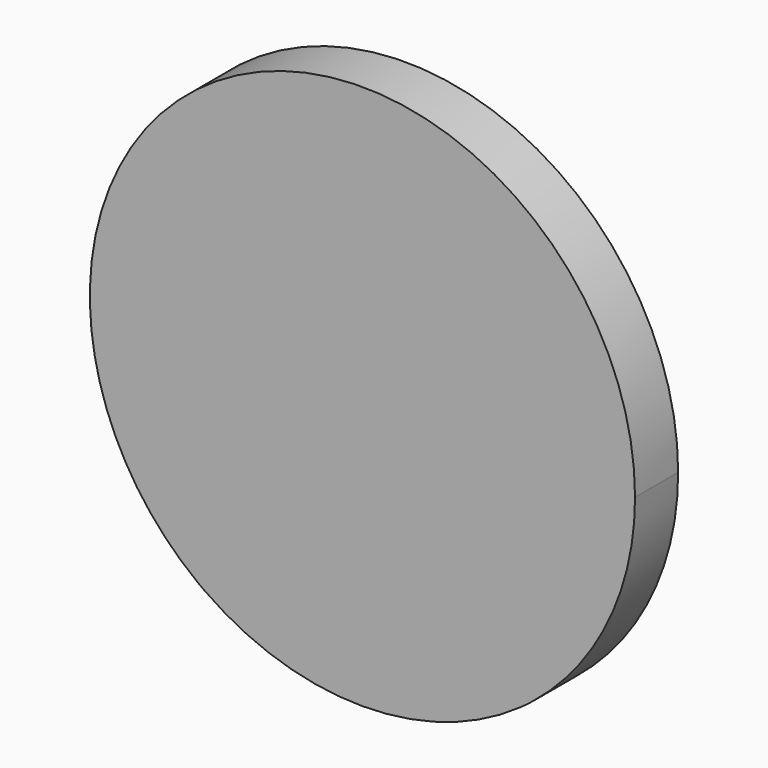
from build123d import *

# Parameters (mm, degrees)
F1_DEPTH = 10


# Not quite as in the source:
# - a feature names something its author has since deleted; it is built from what else it names


with BuildPart() as f1:
    # F0 (on Front) → F1 (new body)
    with BuildSketch(Plane.XZ):
        with BuildLine():
            ThreePointArc((0, 12.4140736889), (4.3797238065, 11.6158187371), (8.1961939537, 9.3237133283))
            Line((8.1961939537, 9.3237133283), (21.0697077151, 23.9681876437))
            ThreePointArc((21.0697077151, 23.9681876437), (18.4530079812, 27.8283575749), (18.0439527664, 32.4738611241))
            Line((18.0439527664, 32.4738611241), (12.5602155062, 33.3932852461))
            Line((12.5602155062, 33.3932852461), (7.5710593451, 36.5340338213))
            ThreePointArc((7.5710593451, 36.5340338213), (4.3242109258, 33.4682836339), (0, 32.3538112298))
            Line((0, 32.3538112298), (0, 12.4140736889))
        make_face()
        with BuildLine():
            ThreePointArc((-7.9262057201, 9.554291624), (-4.2131665816, 11.6772622181), (0, 12.4140736889))
            Line((0, 12.4140736889), (0, 32.3538112298))
            ThreePointArc((0, 32.3538112298), (-4.3563302657, 33.4861038791), (-7.6099407791, 36.5963641019))
            Line((-7.6099407791, 36.5963641019), (-12.278520326, 33.7106778775))
            Line((-12.278520326, 33.7106778775), (-17.78879081, 33.0882026957))
            ThreePointArc((-17.78879081, 33.0882026957), (-17.7466642393, 32.5900633313), (-17.73260723, 32.0903435349))
            ThreePointArc((-17.73260723, 32.0903435349), (-18.5760333574, 28.310954716), (-20.9462636845, 25.2487405378))
            Line((-20.9462636845, 25.2487405378), (-7.9262057201, 9.554291624))
        make_face()
        with BuildLine():
            Line((-12.278520326, 33.7106778775), (-7.6099407791, 36.5963641019))
            ThreePointArc((-7.6099407791, 36.5963641019), (-8.921680068, 41.9636267042), (-6.8304445709, 47.0778130421))
            ThreePointArc((-6.8304445709, 47.0778130421), (-17.0260006599, 47.3423785206), (-24.8514976267, 40.8016632631))
            ThreePointArc((-24.8514976267, 40.8016632631), (-20.0657845476, 38.0934673525), (-17.78879081, 33.0882026957))
            Line((-17.78879081, 33.0882026957), (-12.278520326, 33.7106778775))
        make_face()
        with BuildLine():
            ThreePointArc((-6.8304445709, 47.0778130421), (-8.921680068, 41.9636267042), (-7.6099407791, 36.5963641019))
            Line((-7.6099407791, 36.5963641019), (0, 41.3001291454))
            ThreePointArc((0, 41.3001291454), (-2.9563177988, 44.7314932731), (-6.8304445709, 47.0778130421))
        make_face()
        with BuildLine():
            ThreePointArc((-6.8304445709, 47.0778130421), (-2.9563177988, 44.7314932731), (0, 41.3001291454))
            ThreePointArc((0, 41.3001291454), (2.9670877078, 44.7179968563), (6.8263210631, 47.0826843755))
            ThreePointArc((6.8263210631, 47.0826843755), (-0.0031911285, 50.2464464918), (-6.8304445709, 47.0778130421))
        make_face()
        with BuildLine():
            Line((0, 41.3001291454), (7.5710593451, 36.5340338213))
            ThreePointArc((7.5710593451, 36.5340338213), (8.5956299393, 38.8198569439), (8.9463179156, 41.3001291454))
            ThreePointArc((8.9463179156, 41.3001291454), (8.3996143563, 44.3795906098), (6.8263210631, 47.0826843755))
            ThreePointArc((6.8263210631, 47.0826843755), (2.9670877078, 44.7179968563), (0, 41.3001291454))
        make_face()
        with BuildLine():
            Line((0, 41.3001291454), (0, 32.3538112298))
            ThreePointArc((0, 32.3538112298), (4.3242109258, 33.4682836339), (7.5710593451, 36.5340338213))
            Line((7.5710593451, 36.5340338213), (0, 41.3001291454))
        make_face()
        with BuildLine():
            ThreePointArc((-7.6099407791, 36.5963641019), (-4.3563302657, 33.4861038791), (0, 32.3538112298))
            Line((0, 32.3538112298), (0, 41.3001291454))
            Line((0, 41.3001291454), (-7.6099407791, 36.5963641019))
        make_face()
        with BuildLine():
            ThreePointArc((36.4223056753, 29.9139118839), (45.9083800473, 20.8806963335), (46.4937895072, 7.7947540314))
            ThreePointArc((46.4937895072, 7.7947540314), (49.4692239822, 4.3915233547), (50.5414702125, 0))
            ThreePointArc((50.5414702125, 0), (49.3916524089, -4.5377847699), (46.2196804198, -7.9804821571))
            ThreePointArc((46.2196804198, -7.9804821571), (45.2541028323, -22.5688235592), (34.2624022156, -32.2090809466))
            ThreePointArc((34.2624022156, -32.2090809466), (34.2845647661, -32.5811281227), (34.291956159, -32.953761518))
            ThreePointArc((34.291956159, -32.953761518), (33.6295574849, -36.4193105223), (31.7357494034, -39.3962708606))
            ThreePointArc((31.7357494034, -39.3962708606), (45.6327545118, -21.8374829955), (50.5887729434, 0))
            ThreePointArc((50.5887729434, 0), (0.6523386875, 50.5845668377), (-50.5719492199, 1.3045689002))
            ThreePointArc((-50.5719492199, 1.3045689002), (-49.1901644057, 5.1967911583), (-46.3448391854, 8.1905927165))
            ThreePointArc((-46.3448391854, 8.1905927165), (-45.5368746407, 21.848912941), (-35.4561087337, 31.0998954179))
            ThreePointArc((-35.4561087337, 31.0998954179), (-32.6224058372, 38.6491093328), (-24.8514976267, 40.8016632631))
            ThreePointArc((-24.8514976267, 40.8016632631), (-17.0260006599, 47.3423785206), (-6.8304445709, 47.0778130421))
            ThreePointArc((-6.8304445709, 47.0778130421), (-0.0031911285, 50.2464464918), (6.8263210631, 47.0826843755))
            ThreePointArc((6.8263210631, 47.0826843755), (17.6788975714, 47.324411831), (25.7932452382, 40.1137106881))
            ThreePointArc((25.7932452382, 40.1137106881), (33.2437406928, 37.9811469414), (36.4791003688, 30.9391189367))
            ThreePointArc((36.4791003688, 30.9391189367), (36.4648908183, 30.425729431), (36.4223056753, 29.9139118839))
        make_face()
        with BuildLine():
            ThreePointArc((-46.3448391854, 8.1905927165), (-40.2671562667, 9.9229363025), (-34.3745943291, 7.6388702415))
            Line((-34.3745943291, 7.6388702415), (-29.0687931112, 14.021677727))
            Line((-29.0687931112, 14.021677727), (-27.8149031494, 23.2813171291))
            ThreePointArc((-27.8149031494, 23.2813171291), (-32.9795051289, 25.8770971269), (-35.4561087337, 31.0998954179))
            ThreePointArc((-35.4561087337, 31.0998954179), (-45.5368746407, 21.848912941), (-46.3448391854, 8.1905927165))
        make_face()
        with BuildLine():
            ThreePointArc((-35.4561087337, 31.0998954179), (-32.9795051289, 25.8770971269), (-27.8149031494, 23.2813171291))
            Line((-27.8149031494, 23.2813171291), (-26.6220327467, 32.0903435349))
            ThreePointArc((-26.6220327467, 32.0903435349), (-31.1003542851, 32.1417240723), (-35.4561087337, 31.0998954179))
        make_face()
        with BuildLine():
            ThreePointArc((-35.4561087337, 31.0998954179), (-31.1003542851, 32.1417240723), (-26.6220327467, 32.0903435349))
            ThreePointArc((-26.6220327467, 32.0903435349), (-26.4240541647, 36.5856916795), (-24.8514976267, 40.8016632631))
            ThreePointArc((-24.8514976267, 40.8016632631), (-32.6224058372, 38.6491093328), (-35.4561087337, 31.0998954179))
        make_face()
        with BuildLine():
            ThreePointArc((-24.8514976267, 40.8016632631), (-26.4240541647, 36.5856916795), (-26.6220327467, 32.0903435349))
            Line((-26.6220327467, 32.0903435349), (-17.78879081, 33.0882026957))
            ThreePointArc((-17.78879081, 33.0882026957), (-20.0657845476, 38.0934673525), (-24.8514976267, 40.8016632631))
        make_face()
        with BuildLine():
            Line((-26.6220327467, 32.0903435349), (-20.9462636845, 25.2487405378))
            ThreePointArc((-20.9462636845, 25.2487405378), (-18.5760333574, 28.310954716), (-17.73260723, 32.0903435349))
            ThreePointArc((-17.73260723, 32.0903435349), (-17.7466642393, 32.5900633313), (-17.78879081, 33.0882026957))
            Line((-17.78879081, 33.0882026957), (-26.6220327467, 32.0903435349))
        make_face()
        with BuildLine():
            ThreePointArc((-27.8149031494, 23.2813171291), (-24.1742207002, 23.544578373), (-20.9462636845, 25.2487405378))
            Line((-20.9462636845, 25.2487405378), (-26.6220327467, 32.0903435349))
            Line((-26.6220327467, 32.0903435349), (-27.8149031494, 23.2813171291))
        make_face()
        with BuildLine():
            Line((-30.7910450859, 0), (-12.4140736889, 0))
            ThreePointArc((-12.4140736889, 0), (-11.2362299602, 5.27791264), (-7.9262057201, 9.554291624))
            Line((-7.9262057201, 9.554291624), (-20.9462636845, 25.2487405378))
            ThreePointArc((-20.9462636845, 25.2487405378), (-24.1742207002, 23.544578373), (-27.8149031494, 23.2813171291))
            Line((-27.8149031494, 23.2813171291), (-29.0687931112, 14.021677727))
            Line((-29.0687931112, 14.021677727), (-34.3745943291, 7.6388702415))
            ThreePointArc((-34.3745943291, 7.6388702415), (-31.7314462624, 4.2188317027), (-30.7910450859, 0))
        make_face()
        with BuildLine():
            ThreePointArc((-34.0750304122, -7.3795789352), (-31.6491009662, -4.0386490589), (-30.7910450859, 0))
            Line((-30.7910450859, 0), (-40.7245159149, 0))
            Line((-40.7245159149, 0), (-34.0750304122, -7.3795789352))
        make_face()
        with BuildLine():
            Line((-40.7245159149, 0), (-30.7910450859, 0))
            ThreePointArc((-30.7910450859, 0), (-31.7314462624, 4.2188317027), (-34.3745943291, 7.6388702415))
            Line((-34.3745943291, 7.6388702415), (-40.7245159149, 0))
        make_face()
        with BuildLine():
            Line((-40.7245159149, 0), (-34.3745943291, 7.6388702415))
            ThreePointArc((-34.3745943291, 7.6388702415), (-40.2671562667, 9.9229363025), (-46.3448391854, 8.1905927165))
            ThreePointArc((-46.3448391854, 8.1905927165), (-44.1031958217, 3.7051833857), (-40.7245159149, 0))
        make_face()
        with BuildLine():
            ThreePointArc((-46.139511468, -8.3277647585), (-43.9781949987, -3.8087367386), (-40.7245159149, 0))
            ThreePointArc((-40.7245159149, 0), (-44.1031958217, 3.7051833857), (-46.3448391854, 8.1905927165))
            ThreePointArc((-46.3448391854, 8.1905927165), (-49.1901644057, 5.1967911583), (-50.5719492199, 1.3045689002))
            ThreePointArc((-50.5719492199, 1.3045689002), (-50.5887729434, 0), (-50.5719492199, -1.3045689002))
            ThreePointArc((-50.5719492199, -1.3045689002), (-49.1249179099, -5.3016119279), (-46.139511468, -8.3277647585))
        make_face()
        with BuildLine():
            ThreePointArc((-46.139511468, -8.3277647585), (-39.9462129869, -9.9029332657), (-34.0750304122, -7.3795789352))
            Line((-34.0750304122, -7.3795789352), (-40.7245159149, 0))
            ThreePointArc((-40.7245159149, 0), (-43.9781949987, -3.8087367386), (-46.139511468, -8.3277647585))
        make_face()
        with BuildLine():
            ThreePointArc((-30.5009303557, -40.3598463247), (-33.0177016325, -36.8777345609), (-33.7279636415, -32.640427884))
            ThreePointArc((-33.7279636415, -32.640427884), (-44.9854308164, -23.0629718726), (-46.139511468, -8.3277647585))
            ThreePointArc((-46.139511468, -8.3277647585), (-49.1249179099, -5.3016119279), (-50.5719492199, -1.3045689002))
            ThreePointArc((-50.5719492199, -1.3045689002), (-44.9947955251, -23.1234150499), (-30.5009303557, -40.3598463247))
        make_face()
        with BuildLine():
            ThreePointArc((-33.7279636415, -32.640427884), (-31.3725828689, -26.9858355888), (-26.0396213441, -23.9722407284))
            Line((-26.0396213441, -23.9722407284), (-27.8331619734, -14.3067856835))
            Line((-27.8331619734, -14.3067856835), (-34.0750304122, -7.3795789352))
            ThreePointArc((-34.0750304122, -7.3795789352), (-39.9462129869, -9.9029332657), (-46.139511468, -8.3277647585))
            ThreePointArc((-46.139511468, -8.3277647585), (-44.9854308164, -23.0629718726), (-33.7279636415, -32.640427884))
        make_face()
        with BuildLine():
            Line((-18.7530413406, -25.632855502), (-7.3299455485, -10.0190380681))
            ThreePointArc((-7.3299455485, -10.0190380681), (-11.0703141267, -5.6175947424), (-12.4140736889, 0))
            Line((-12.4140736889, 0), (-30.7910450859, 0))
            ThreePointArc((-30.7910450859, 0), (-31.6491009662, -4.0386490589), (-34.0750304122, -7.3795789352))
            Line((-34.0750304122, -7.3795789352), (-27.8331619734, -14.3067856835))
            Line((-27.8331619734, -14.3067856835), (-26.0396213441, -23.9722407284))
            ThreePointArc((-26.0396213441, -23.9722407284), (-22.2247546471, -24.0496899951), (-18.7530413406, -25.632855502))
        make_face()
        with BuildLine():
            Line((-24.3195872754, -33.2415662706), (-18.7530413406, -25.632855502))
            ThreePointArc((-18.7530413406, -25.632855502), (-22.2247546471, -24.0496899951), (-26.0396213441, -23.9722407284))
            Line((-26.0396213441, -23.9722407284), (-24.3195872754, -33.2415662706))
        make_face()
        with BuildLine():
            Line((-24.3195872754, -33.2415662706), (-26.0396213441, -23.9722407284))
            ThreePointArc((-26.0396213441, -23.9722407284), (-31.3725828689, -26.9858355888), (-33.7279636415, -32.640427884))
            ThreePointArc((-33.7279636415, -32.640427884), (-29.0611287118, -33.5256103283), (-24.3195872754, -33.2415662706))
        make_face()
        with BuildLine():
            ThreePointArc((-22.7066374003, -42.5301240653), (-24.4011253438, -38.0400478438), (-24.3195872754, -33.2415662706))
            ThreePointArc((-24.3195872754, -33.2415662706), (-29.0611287118, -33.5256103283), (-33.7279636415, -32.640427884))
            ThreePointArc((-33.7279636415, -32.640427884), (-33.0177016325, -36.8777345609), (-30.5009303557, -40.3598463247))
            ThreePointArc((-30.5009303557, -40.3598463247), (-29.8703681269, -40.8287283157), (-29.2325991317, -41.2877596379))
            ThreePointArc((-29.2325991317, -41.2877596379), (-26.0826725293, -42.5027996438), (-22.7066374003, -42.5301240653))
        make_face()
        with BuildLine():
            Line((-15.0911921565, -35.1691649674), (-24.3195872754, -33.2415662706))
            ThreePointArc((-24.3195872754, -33.2415662706), (-24.4011253438, -38.0400478438), (-22.7066374003, -42.5301240653))
            ThreePointArc((-22.7066374003, -42.5301240653), (-17.7675173712, -40.0201570663), (-15.0911921565, -35.1691649674))
        make_face()
        with BuildLine():
            ThreePointArc((-14.8920259149, -33.2415662706), (-15.9125108938, -28.9754228225), (-18.7530413406, -25.632855502))
            Line((-18.7530413406, -25.632855502), (-24.3195872754, -33.2415662706))
            Line((-24.3195872754, -33.2415662706), (-15.0911921565, -35.1691649674))
            ThreePointArc((-15.0911921565, -35.1691649674), (-14.9419496612, -34.2104965993), (-14.8920259149, -33.2415662706))
        make_face()
        with BuildLine():
            Line((0, -31.5046176402), (0, -12.4140736889))
            ThreePointArc((0, -12.4140736889), (-3.8556548526, -11.8001335252), (-7.3299455485, -10.0190380681))
            Line((-7.3299455485, -10.0190380681), (-18.7530413406, -25.632855502))
            ThreePointArc((-18.7530413406, -25.632855502), (-15.9125108938, -28.9754228225), (-14.8920259149, -33.2415662706))
            ThreePointArc((-14.8920259149, -33.2415662706), (-14.9419496612, -34.2104965993), (-15.0911921565, -35.1691649674))
            Line((-15.0911921565, -35.1691649674), (-11.8124056821, -35.854027769))
            Line((-11.8124056821, -35.854027769), (-8.5237688791, -37.209996633))
            ThreePointArc((-8.5237688791, -37.209996633), (-5.1284984488, -33.0625960348), (0, -31.5046176402))
        make_face()
        with BuildLine():
            ThreePointArc((-6.3531457642, -47.4061283415), (-9.0178114186, -42.6442863227), (-8.5237688791, -37.209996633))
            Line((-8.5237688791, -37.209996633), (-11.8124056821, -35.854027769))
            Line((-11.8124056821, -35.854027769), (-15.0911921565, -35.1691649674))
            ThreePointArc((-15.0911921565, -35.1691649674), (-17.7675173712, -40.0201570663), (-22.7066374003, -42.5301240653))
            ThreePointArc((-22.7066374003, -42.5301240653), (-15.4632390175, -48.0984535393), (-6.3531457642, -47.4061283415))
        make_face()
        with BuildLine():
            ThreePointArc((29.2228790167, -41.2946399656), (26.2897143388, -42.2464687444), (23.206366099, -42.197512799))
            ThreePointArc((23.206366099, -42.197512799), (15.8115613872, -47.9336831156), (6.4750778857, -47.288034253))
            ThreePointArc((6.4750778857, -47.288034253), (0.0848729286, -49.9440160857), (-6.3531457642, -47.4061283415))
            ThreePointArc((-6.3531457642, -47.4061283415), (-15.4632390175, -48.0984535393), (-22.7066374003, -42.5301240653))
            ThreePointArc((-22.7066374003, -42.5301240653), (-26.0826725293, -42.5027996438), (-29.2325991317, -41.2877596379))
            ThreePointArc((-29.2325991317, -41.2877596379), (-0.0059544006, -50.588772593), (29.2228790167, -41.2946399656))
        make_face()
        with BuildLine():
            Line((19.2309829091, -25.4560439964), (7.4830019114, -9.905246486))
            ThreePointArc((7.4830019114, -9.905246486), (3.9461858655, -11.7701674869), (0, -12.4140736889))
            Line((0, -12.4140736889), (0, -31.5046176402))
            ThreePointArc((0, -31.5046176402), (5.0176698122, -32.9895625997), (8.4190600767, -36.9660706339))
            Line((8.4190600767, -36.9660706339), (11.9896721342, -35.3720759819))
            Line((11.9896721342, -35.3720759819), (15.6591926585, -34.6844592594))
            ThreePointArc((15.6591926585, -34.6844592594), (16.1319190758, -29.5619993381), (19.2309829091, -25.4560439964))
        make_face()
        with BuildLine():
            ThreePointArc((23.206366099, -42.197512799), (18.2657550813, -39.6133102694), (15.6591926585, -34.6844592594))
            Line((15.6591926585, -34.6844592594), (11.9896721342, -35.3720759819))
            Line((11.9896721342, -35.3720759819), (8.4190600767, -36.9660706339))
            ThreePointArc((8.4190600767, -36.9660706339), (9.0174636571, -38.8031052324), (9.2198945494, -40.7245121896))
            ThreePointArc((9.2198945494, -40.7245121896), (8.5060563956, -44.2816824271), (6.4750778857, -47.288034253))
            ThreePointArc((6.4750778857, -47.288034253), (15.8115613872, -47.9336831156), (23.206366099, -42.197512799))
        make_face()
        with BuildLine():
            ThreePointArc((8.4190600767, -36.9660706339), (5.0176698122, -32.9895625997), (0, -31.5046176402))
            Line((0, -31.5046176402), (0, -40.7245121896))
            Line((0, -40.7245121896), (8.4190600767, -36.9660706339))
        make_face()
        with BuildLine():
            Line((0, -40.7245121896), (0, -31.5046176402))
            ThreePointArc((0, -31.5046176402), (-5.1284984488, -33.0625960348), (-8.5237688791, -37.209996633))
            Line((-8.5237688791, -37.209996633), (0, -40.7245121896))
        make_face()
        with BuildLine():
            Line((0, -40.7245121896), (-8.5237688791, -37.209996633))
            ThreePointArc((-8.5237688791, -37.209996633), (-9.0178114186, -42.6442863227), (-6.3531457642, -47.4061283415))
            ThreePointArc((-6.3531457642, -47.4061283415), (-2.5528912915, -44.6583414697), (0, -40.7245121896))
        make_face()
        with BuildLine():
            ThreePointArc((6.4750778857, -47.288034253), (2.6424912294, -44.5933026018), (0, -40.7245121896))
            ThreePointArc((0, -40.7245121896), (-2.5528912915, -44.6583414697), (-6.3531457642, -47.4061283415))
            ThreePointArc((-6.3531457642, -47.4061283415), (0.0848729286, -49.9440160857), (6.4750778857, -47.288034253))
        make_face()
        with BuildLine():
            ThreePointArc((9.2198945494, -40.7245121896), (9.0174636571, -38.8031052324), (8.4190600767, -36.9660706339))
            Line((8.4190600767, -36.9660706339), (0, -40.7245121896))
            ThreePointArc((0, -40.7245121896), (2.6424912294, -44.5933026018), (6.4750778857, -47.288034253))
            ThreePointArc((6.4750778857, -47.288034253), (8.5060563956, -44.2816824271), (9.2198945494, -40.7245121896))
        make_face()
        with BuildLine():
            Line((31.4831711226, 0), (12.4140736889, 0))
            ThreePointArc((12.4140736889, 0), (11.113140031, -5.5323904603), (7.4830019114, -9.905246486))
            Line((7.4830019114, -9.905246486), (19.2309829091, -25.4560439964))
            ThreePointArc((19.2309829091, -25.4560439964), (22.6706111136, -23.8241226738), (26.4754028959, -23.6908227053))
            Line((26.4754028959, -23.6908227053), (28.1101843832, -14.1079709863))
            Line((28.1101843832, -14.1079709863), (34.5814156225, -7.0319379514))
            ThreePointArc((34.5814156225, -7.0319379514), (32.2920641652, -3.8421110842), (31.4831711226, 0))
        make_face()
        with BuildLine():
            ThreePointArc((46.2196804198, -7.9804821571), (40.2382406985, -9.4976571454), (34.5814156225, -7.0319379514))
            Line((34.5814156225, -7.0319379514), (28.1101843832, -14.1079709863))
            Line((28.1101843832, -14.1079709863), (26.4754028959, -23.6908227053))
            ThreePointArc((26.4754028959, -23.6908227053), (31.8307310628, -26.6136155389), (34.2624022156, -32.2090809466))
            ThreePointArc((34.2624022156, -32.2090809466), (45.2541028323, -22.5688235592), (46.2196804198, -7.9804821571))
        make_face()
        with BuildLine():
            ThreePointArc((8.1961939537, 9.3237133283), (11.3105566013, 5.1166917947), (12.4140736889, 0))
            Line((12.4140736889, 0), (31.4831711226, 0))
            ThreePointArc((31.4831711226, 0), (32.4069275416, 4.0929085256), (34.9990987759, 7.3922833775))
            Line((34.9990987759, 7.3922833775), (29.9410622795, 13.6103208604))
            Line((29.9410622795, 13.6103208604), (28.6489670456, 21.7718335631))
            ThreePointArc((28.6489670456, 21.7718335631), (24.6142989754, 22.0244230757), (21.0697077151, 23.9681876437))
            Line((21.0697077151, 23.9681876437), (8.1961939537, 9.3237133283))
        make_face()
        with BuildLine():
            Line((12.5602155062, 33.3932852461), (18.0439527664, 32.4738611241))
            ThreePointArc((18.0439527664, 32.4738611241), (20.681498993, 37.5486077071), (25.7932452382, 40.1137106881))
            ThreePointArc((25.7932452382, 40.1137106881), (17.6788975714, 47.324411831), (6.8263210631, 47.0826843755))
            ThreePointArc((6.8263210631, 47.0826843755), (8.3996143563, 44.3795906098), (8.9463179156, 41.3001291454))
            ThreePointArc((8.9463179156, 41.3001291454), (8.5956299393, 38.8198569439), (7.5710593451, 36.5340338213))
            Line((7.5710593451, 36.5340338213), (12.5602155062, 33.3932852461))
        make_face()
        with BuildLine():
            ThreePointArc((26.4754028959, -23.6908227053), (22.6706111136, -23.8241226738), (19.2309829091, -25.4560439964))
            Line((19.2309829091, -25.4560439964), (24.8951967806, -32.953761518))
            Line((24.8951967806, -32.953761518), (26.4754028959, -23.6908227053))
        make_face()
        with BuildLine():
            Line((24.8951967806, -32.953761518), (19.2309829091, -25.4560439964))
            ThreePointArc((19.2309829091, -25.4560439964), (16.1319190758, -29.5619993381), (15.6591926585, -34.6844592594))
            Line((15.6591926585, -34.6844592594), (24.8951967806, -32.953761518))
        make_face()
        with BuildLine():
            ThreePointArc((34.2624022156, -32.2090809466), (31.8307310628, -26.6136155389), (26.4754028959, -23.6908227053))
            Line((26.4754028959, -23.6908227053), (24.8951967806, -32.953761518))
            ThreePointArc((24.8951967806, -32.953761518), (29.6252644616, -33.1658958053), (34.2624022156, -32.2090809466))
        make_face()
        with BuildLine():
            ThreePointArc((46.4937895072, 7.7947540314), (44.2923929818, 3.5181009217), (41.0123206675, 0))
            ThreePointArc((41.0123206675, 0), (44.1211918052, -3.6605977574), (46.2196804198, -7.9804821571))
            ThreePointArc((46.2196804198, -7.9804821571), (49.3916524089, -4.5377847699), (50.5414702125, 0))
            ThreePointArc((50.5414702125, 0), (49.4692239822, 4.3915233547), (46.4937895072, 7.7947540314))
        make_face()
        with BuildLine():
            Line((41.0123206675, 0), (34.5814156225, -7.0319379514))
            ThreePointArc((34.5814156225, -7.0319379514), (40.2382406985, -9.4976571454), (46.2196804198, -7.9804821571))
            ThreePointArc((46.2196804198, -7.9804821571), (44.1211918052, -3.6605977574), (41.0123206675, 0))
        make_face()
        with BuildLine():
            ThreePointArc((46.4937895072, 7.7947540314), (40.678875044, 9.523313765), (34.9990987759, 7.3922833775))
            Line((34.9990987759, 7.3922833775), (41.0123206675, 0))
            ThreePointArc((41.0123206675, 0), (44.2923929818, 3.5181009217), (46.4937895072, 7.7947540314))
        make_face()
        with BuildLine():
            Line((29.9410622795, 13.6103208604), (34.9990987759, 7.3922833775))
            ThreePointArc((34.9990987759, 7.3922833775), (40.678875044, 9.523313765), (46.4937895072, 7.7947540314))
            ThreePointArc((46.4937895072, 7.7947540314), (45.9083800473, 20.8806963335), (36.4223056753, 29.9139118839))
            ThreePointArc((36.4223056753, 29.9139118839), (33.9108785019, 24.5299127589), (28.6489670456, 21.7718335631))
            Line((28.6489670456, 21.7718335631), (29.9410622795, 13.6103208604))
        make_face()
        with BuildLine():
            Line((24.8951967806, -32.953761518), (15.6591926585, -34.6844592594))
            ThreePointArc((15.6591926585, -34.6844592594), (18.2657550813, -39.6133102694), (23.206366099, -42.197512799))
            ThreePointArc((23.206366099, -42.197512799), (24.9060219327, -37.7318893488), (24.8951967806, -32.953761518))
        make_face()
        with BuildLine():
            ThreePointArc((34.2624022156, -32.2090809466), (29.6252644616, -33.1658958053), (24.8951967806, -32.953761518))
            ThreePointArc((24.8951967806, -32.953761518), (24.9060219327, -37.7318893488), (23.206366099, -42.197512799))
            ThreePointArc((23.206366099, -42.197512799), (26.2897143388, -42.2464687444), (29.2228790167, -41.2946399656))
            ThreePointArc((29.2228790167, -41.2946399656), (30.494090346, -40.3650145781), (31.7357494034, -39.3962708606))
            ThreePointArc((31.7357494034, -39.3962708606), (33.6295574849, -36.4193105223), (34.291956159, -32.953761518))
            ThreePointArc((34.291956159, -32.953761518), (34.2845647661, -32.5811281227), (34.2624022156, -32.2090809466))
        make_face()
        with BuildLine():
            ThreePointArc((34.9990987759, 7.3922833775), (32.4069275416, 4.0929085256), (31.4831711226, 0))
            Line((31.4831711226, 0), (41.0123206675, 0))
            Line((41.0123206675, 0), (34.9990987759, 7.3922833775))
        make_face()
        with BuildLine():
            Line((41.0123206675, 0), (31.4831711226, 0))
            ThreePointArc((31.4831711226, 0), (32.2920641652, -3.8421110842), (34.5814156225, -7.0319379514))
            Line((34.5814156225, -7.0319379514), (41.0123206675, 0))
        make_face()
        with BuildLine():
            ThreePointArc((25.7932452382, 40.1137106881), (20.681498993, 37.5486077071), (18.0439527664, 32.4738611241))
            Line((18.0439527664, 32.4738611241), (27.1976422518, 30.9391189367))
            ThreePointArc((27.1976422518, 30.9391189367), (27.2310665217, 35.6390199788), (25.7932452382, 40.1137106881))
        make_face()
        with BuildLine():
            ThreePointArc((25.7932452382, 40.1137106881), (27.2310665217, 35.6390199788), (27.1976422518, 30.9391189367))
            ThreePointArc((27.1976422518, 30.9391189367), (31.8789975875, 31.0475799041), (36.4223056753, 29.9139118839))
            ThreePointArc((36.4223056753, 29.9139118839), (36.4648908183, 30.425729431), (36.4791003688, 30.9391189367))
            ThreePointArc((36.4791003688, 30.9391189367), (33.2437406928, 37.9811469414), (25.7932452382, 40.1137106881))
        make_face()
        with BuildLine():
            Line((27.1976422518, 30.9391189367), (28.6489670456, 21.7718335631))
            ThreePointArc((28.6489670456, 21.7718335631), (33.9108785019, 24.5299127589), (36.4223056753, 29.9139118839))
            ThreePointArc((36.4223056753, 29.9139118839), (31.8789975875, 31.0475799041), (27.1976422518, 30.9391189367))
        make_face()
        with BuildLine():
            Line((27.1976422518, 30.9391189367), (21.0697077151, 23.9681876437))
            ThreePointArc((21.0697077151, 23.9681876437), (24.6142989754, 22.0244230757), (28.6489670456, 21.7718335631))
            Line((28.6489670456, 21.7718335631), (27.1976422518, 30.9391189367))
        make_face()
        with BuildLine():
            ThreePointArc((18.0439527664, 32.4738611241), (18.4530079812, 27.8283575749), (21.0697077151, 23.9681876437))
            Line((21.0697077151, 23.9681876437), (27.1976422518, 30.9391189367))
            Line((27.1976422518, 30.9391189367), (18.0439527664, 32.4738611241))
        make_face()
        with BuildLine():
            Line((0, 0), (8.1961939537, 9.3237133283))
            ThreePointArc((8.1961939537, 9.3237133283), (4.3797238065, 11.6158187371), (0, 12.4140736889))
            Line((0, 12.4140736889), (0, 0))
        make_face()
        with BuildLine():
            Line((-7.9262057201, 9.554291624), (0, 0))
            Line((0, 0), (0, 12.4140736889))
            ThreePointArc((0, 12.4140736889), (-4.2131665816, 11.6772622181), (-7.9262057201, 9.554291624))
        make_face()
        with BuildLine():
            Line((-12.4140736889, 0), (0, 0))
            Line((0, 0), (-7.9262057201, 9.554291624))
            ThreePointArc((-7.9262057201, 9.554291624), (-11.2362299602, 5.27791264), (-12.4140736889, 0))
        make_face()
        with BuildLine():
            Line((-7.3299455485, -10.0190380681), (0, 0))
            Line((0, 0), (-12.4140736889, 0))
            ThreePointArc((-12.4140736889, 0), (-11.0703141267, -5.6175947424), (-7.3299455485, -10.0190380681))
        make_face()
        with BuildLine():
            Line((0, -12.4140736889), (0, 0))
            Line((0, 0), (-7.3299455485, -10.0190380681))
            ThreePointArc((-7.3299455485, -10.0190380681), (-3.8556548526, -11.8001335252), (0, -12.4140736889))
        make_face()
        with BuildLine():
            ThreePointArc((0, -12.4140736889), (3.9461858655, -11.7701674869), (7.4830019114, -9.905246486))
            Line((7.4830019114, -9.905246486), (0, 0))
            Line((0, 0), (0, -12.4140736889))
        make_face()
        with BuildLine():
            ThreePointArc((7.4830019114, -9.905246486), (11.113140031, -5.5323904603), (12.4140736889, 0))
            Line((12.4140736889, 0), (0, 0))
            Line((0, 0), (7.4830019114, -9.905246486))
        make_face()
        with BuildLine():
            Line((0, 0), (12.4140736889, 0))
            ThreePointArc((12.4140736889, 0), (11.3105566013, 5.1166917947), (8.1961939537, 9.3237133283))
            Line((8.1961939537, 9.3237133283), (0, 0))
        make_face()
    extrude(amount=F1_DEPTH)


solid = f1.part
